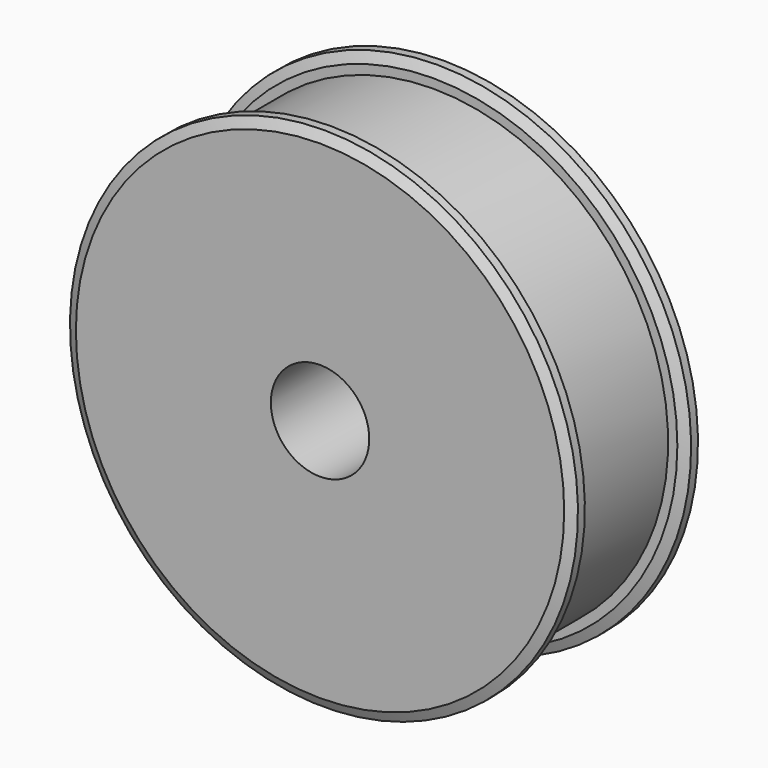
from build123d import *

# Parameters (mm, degrees)
F2_C1_SIZE2 = 0.4
F2_C1_SIZE  = 0.8
F2_C2_SIZE2 = 0.8
F2_C2_SIZE  = 0.4
F2_C3_SIZE2 = 0.8
F2_C3_SIZE  = 0.4
F3_SIZE2    = 0.4
F3_SIZE     = 0.8
F4_SIZE     = 0.4


with BuildPart() as f1:
    # F0 (on Right) → F1 (revolve)
    with BuildSketch(Plane.YZ):
        Polygon((-10.3, 20.65), (-10.3, 4), (10.3, 4), (10.3, 9.55), (3.2, 9.55), (3.2, 6.35), (2.7, 6.35), (2.7, 20.65), (1.2, 20.65), (1.2, 19.1), (-8.8, 19.1), (-8.8, 20.65), align=None)
    revolve(axis=Axis((0, -3.1587743408, 0), (0, -1, 0)))

    # F2: chamfer of 0.4 x 0.8 on 3 edges, made by hand

    # F2_c1
    f2_c1_edges = [f1.edges().sort_by_distance(p)[0] for p in [
        (0, -10.3, -20.65),
    ]]
    f2_c1_side = f1.faces().sort_by_distance((0, -10.3, -20.642))[0]
    chamfer(f2_c1_edges, length=F2_C1_SIZE, length2=F2_C1_SIZE2, reference=f2_c1_side)

    # F2_c2
    f2_c2_edges = [f1.edges().sort_by_distance(p)[0] for p in [
        (0, 2.7, -20.65),
    ]]
    f2_c2_side = f1.faces().sort_by_distance((0, 2.692, -20.65))[0]
    chamfer(f2_c2_edges, length=F2_C2_SIZE, length2=F2_C2_SIZE2, reference=f2_c2_side)

    # F2_c3
    f2_c3_edges = [f1.edges().sort_by_distance(p)[0] for p in [
        (0, 1.2, -20.65),
    ]]
    f2_c3_side = f1.faces().sort_by_distance((0, 1.208, -20.65))[0]
    chamfer(f2_c3_edges, length=F2_C3_SIZE, length2=F2_C3_SIZE2, reference=f2_c3_side)

    # F3
    f3_edges = [f1.edges().sort_by_distance(p)[0] for p in [
        (0, -8.8, -20.65),
    ]]
    chamfer(f3_edges, length=F3_SIZE, length2=F3_SIZE2)

    # F4
    f4_edges = [f1.edges().sort_by_distance(p)[0] for p in [
        (0, 3.2, -9.55),
        (0, 10.3, -9.55),
    ]]
    chamfer(f4_edges, length=F4_SIZE)


solid = f1.part
